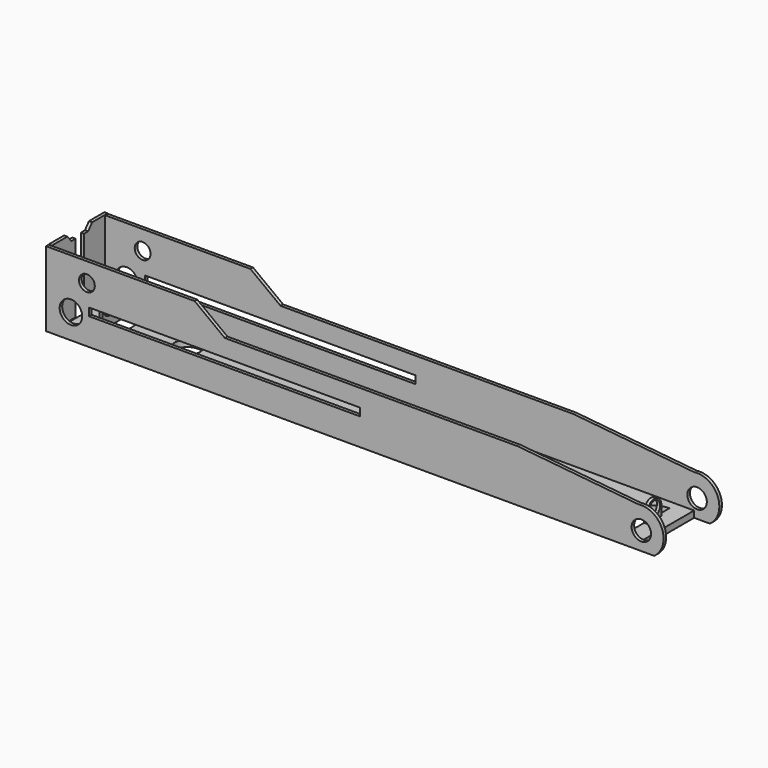
from build123d import *

# Parameters (mm, degrees)
F0_R      = 1.75
F0_R_2    = 1.51
F0_R_3    = 1.225
F8_DEPTH  = 0.5
F2_R      = 1.75
F2_R_2    = 1.51
F2_R_3    = 1.225
F9_DEPTH  = 0.5
F7_R      = 1.97
F10_DEPTH = 0.5
F11_DEPTH = 1
F12_DEPTH = 0.5
F13_DEPTH = 25
F16_DEPTH = 0.5
F17_DEPTH = 0.5
F18_W     = 41.976
F18_H     = 1.2
F19_DEPTH = 11.301


# Not quite as in the source:
# - a feature names something its author has since deleted; it is built from what else it names


with BuildPart() as f8:
    # F0 (on Front) → F8 (new body)
    with BuildSketch(Plane.XZ):
        with BuildLine():
            Line((-24.095, 11.6), (-47.125, 11.6))
            Line((-47.125, 11.6), (-47.125, 0))
            Line((-47.125, 0), (47.125, 0))
            ThreePointArc((47.125, 0), (48.3457892371, 4.0785044966), (44.6764603032, 6.2373353065))
            Line((44.6764603032, 6.2373353065), (25.9870177338, 8.0793821146))
            Line((25.9870177338, 8.0793821146), (-19.4229822662, 8.0793821146))
            Line((-19.4229822662, 8.0793821146), (-24.095, 11.6))
        make_face()
        with Locations((-43.275, 3.85)):
            Circle(F0_R, mode=Mode.SUBTRACT)
        with Locations((45.1343327214, 2.8178092836)):
            Circle(F0_R_2, mode=Mode.SUBTRACT)
        with Locations((-40.8, 8.615)):
            Circle(F0_R_3, mode=Mode.SUBTRACT)
    extrude(amount=F8_DEPTH)

    # F6 (on offset) → F9, piece 2 (join)
    with BuildSketch(Plane.YZ.offset(-47.125)):
        Polygon((3.7804580054, 10.7198863682), (3, 11.65), (0, 11.65), (0, 0), (4.5804580054, 0), (4.5804580054, 10.7198863682), align=None)
    extrude(amount=F9_DEPTH)



with BuildPart() as f8b:
    # F2 (on offset) → F8, piece 2 (new body)
    with BuildSketch(Plane.XZ.offset(-10.8)):
        with BuildLine():
            Line((-19.4229822662, 8.0793821146), (-24.095, 11.6))
            Line((-24.095, 11.6), (-47.125, 11.6))
            Line((-47.125, 11.6), (-47.125, 0))
            Line((-47.125, 0), (47.125, 0))
            ThreePointArc((47.125, 0), (48.3457892371, 4.0785044966), (44.6764603032, 6.2373353065))
            Line((44.6764603032, 6.2373353065), (25.9870177338, 8.0793821146))
            Line((25.9870177338, 8.0793821146), (-19.4229822662, 8.0793821146))
        make_face()
        with Locations((-43.275, 3.85)):
            Circle(F2_R, mode=Mode.SUBTRACT)
        with Locations((45.1343327214, 2.8178092836)):
            Circle(F2_R_2, mode=Mode.SUBTRACT)
        with Locations((-40.8, 8.615)):
            Circle(F2_R_3, mode=Mode.SUBTRACT)
    extrude(amount=F8_DEPTH)

    # F6 (on offset) → F9 (join)
    with BuildSketch(Plane.YZ.offset(-47.125)):
        Polygon((10.8, 0), (10.8, 11.65), (7.8, 11.65), (7.0195419946, 10.7198863682), (6.2195419946, 10.7198863682), (6.2195419946, 0), align=None)
    extrude(amount=F9_DEPTH)


with BuildPart() as f8_1:
    add(f8.part)

    add(f8b.part)  # F10 merges F8b
    # F7 (on Top) → F10 (join)
    with BuildSketch(Plane.XY):
        Polygon((-47.125, 4.45), (-47.125, 0), (-46.325, 0), (-46.325, 1.5), (-45.2581904829, 1.5), (-45.2581904829, 9.3), (-46.325, 9.3), (-46.325, 10.8), (-47.125, 10.8), (-47.125, 5.95), align=None)
        Polygon((-46.325, 1.5), (-46.325, 0), (-24.095, 0), (-19.4229822662, 0), (25.9870177338, 0), (44.676, 0), (44.676, 10.8), (25.9870177338, 10.8), (-19.4229822662, 10.8), (-46.325, 10.8), (-46.325, 9.3), (-45.2581904829, 9.3), (-45.2581904829, 1.5), align=None)
        with BuildLine():
            Line((-41.976, 1.89), (-41.976, 8.91))
            ThreePointArc((-41.976, 8.91), (-38.466, 5.4), (-41.976, 1.89))
        make_face(mode=Mode.SUBTRACT)
        with Locations((-29.946, 5.4)):
            Circle(F7_R, mode=Mode.SUBTRACT)
        with Locations((29.946, 5.4)):
            Circle(F7_R, mode=Mode.SUBTRACT)
        with BuildLine():
            Line((41.976, 8.91), (41.976, 1.89))
            ThreePointArc((41.976, 1.89), (38.466, 5.4), (41.976, 8.91))
        make_face(mode=Mode.SUBTRACT)
    extrude(amount=F10_DEPTH)

    # F7 (on Top) → F11 (join)
    with BuildSketch(Plane.XY):
        Polygon((-46.325, 1.5), (-46.325, 0), (-24.095, 0), (-19.4229822662, 0), (25.9870177338, 0), (44.676, 0), (44.676, 10.8), (25.9870177338, 10.8), (-19.4229822662, 10.8), (-46.325, 10.8), (-46.325, 9.3), (-45.2581904829, 9.3), (-45.2581904829, 1.5), align=None)
        with BuildLine():
            Line((-41.976, 1.89), (-41.976, 8.91))
            ThreePointArc((-41.976, 8.91), (-38.466, 5.4), (-41.976, 1.89))
        make_face(mode=Mode.SUBTRACT)
        with Locations((-29.946, 5.4)):
            Circle(F7_R, mode=Mode.SUBTRACT)
        with Locations((29.946, 5.4)):
            Circle(F7_R, mode=Mode.SUBTRACT)
        with BuildLine():
            Line((41.976, 8.91), (41.976, 1.89))
            ThreePointArc((41.976, 1.89), (38.466, 5.4), (41.976, 8.91))
        make_face(mode=Mode.SUBTRACT)
    extrude(amount=F11_DEPTH)

    # F6 (on offset) → F12 (join)
    with BuildSketch(Plane.YZ.offset(-47.125)):
        Polygon((3.7804580054, 10.7198863682), (3, 11.65), (0, 11.65), (0, 0), (4.5804580054, 0), (4.5804580054, 10.7198863682), align=None)
    extrude(amount=F12_DEPTH)

    # F13 (cut): a face of the model
    f13_faces = [f8_1.faces().sort_by_distance(p)[0] for p in [
        (-46.0368491628, 5.3368390391, 0.5),
    ]]
    extrude(f13_faces, amount=-F13_DEPTH, mode=Mode.SUBTRACT)

    # F14 (on face) → F16 (join)
    with BuildSketch(Plane.YZ.offset(-41.976)):
        with BuildLine():
            Line((4, 2.55), (4, 1))
            Line((4, 1), (4.5804580054, 1))
            Line((4.5804580054, 1), (4.5804580054, 1.7362401346))
            ThreePointArc((4.5804580054, 1.7362401346), (4.23, 2.55), (4.5804580054, 3.3637598654))
            Line((4.5804580054, 3.3637598654), (4.5804580054, 3.6591912001))
            ThreePointArc((4.5804580054, 3.6591912001), (4.1538851032, 3.175946606), (4, 2.55))
        make_face()
        with BuildLine():
            ThreePointArc((6.2195419946, 3.5826648631), (5.4129608614, 3.8985310267), (4.5804580054, 3.6591912001))
            Line((4.5804580054, 3.6591912001), (4.5804580054, 3.3637598654))
            ThreePointArc((4.5804580054, 3.3637598654), (5.4235415848, 3.6675829434), (6.2195419946, 3.2559013526))
            Line((6.2195419946, 3.2559013526), (6.2195419946, 3.5826648631))
        make_face()
        with BuildLine():
            Line((4.5804580054, 1.7362401346), (4.5804580054, 1))
            Line((4.5804580054, 1), (6.2195419946, 1))
            Line((6.2195419946, 1), (6.2195419946, 1.8440986474))
            ThreePointArc((6.2195419946, 1.8440986474), (5.4235415848, 1.4324170566), (4.5804580054, 1.7362401346))
        make_face()
        with BuildLine():
            Line((6.2195419946, 1.8440986474), (6.2195419946, 1))
            Line((6.2195419946, 1), (6.7, 1))
            Line((6.7, 1), (6.7, 2.55))
            ThreePointArc((6.7, 2.55), (6.5740060647, 3.1194814779), (6.2195419946, 3.5826648631))
            Line((6.2195419946, 3.5826648631), (6.2195419946, 3.2559013526))
            ThreePointArc((6.2195419946, 3.2559013526), (6.4055299697, 2.9245083217), (6.47, 2.55))
            ThreePointArc((6.47, 2.55), (6.4055299697, 2.1754916783), (6.2195419946, 1.8440986474))
        make_face()
    extrude(amount=-F16_DEPTH)

    # F15 (on face) → F17 (join)
    with BuildSketch(Plane(origin=(41.976, 0, 0), x_dir=(0, -1, 0), z_dir=(-1, 0, 0))):
        with BuildLine():
            ThreePointArc((-4.5804580054, 3.3637598654), (-4.23, 2.55), (-4.5804580054, 1.7362401346))
            Line((-4.5804580054, 1.7362401346), (-4.5804580054, 1))
            Line((-4.5804580054, 1), (-4, 1))
            Line((-4, 1), (-4, 2.55))
            ThreePointArc((-4, 2.55), (-4.1538851032, 3.175946606), (-4.5804580054, 3.6591912001))
            Line((-4.5804580054, 3.6591912001), (-4.5804580054, 3.3637598654))
        make_face()
        with BuildLine():
            Line((-6.2195419946, 3.5826648631), (-6.2195419946, 3.2559013526))
            ThreePointArc((-6.2195419946, 3.2559013526), (-5.4235415848, 3.6675829434), (-4.5804580054, 3.3637598654))
            Line((-4.5804580054, 3.3637598654), (-4.5804580054, 3.6591912001))
            ThreePointArc((-4.5804580054, 3.6591912001), (-5.4129608614, 3.8985310267), (-6.2195419946, 3.5826648631))
        make_face()
        with BuildLine():
            Line((-6.2195419946, 1), (-6.2195419946, 1.8440986474))
            ThreePointArc((-6.2195419946, 1.8440986474), (-6.47, 2.55), (-6.2195419946, 3.2559013526))
            Line((-6.2195419946, 3.2559013526), (-6.2195419946, 3.5826648631))
            ThreePointArc((-6.2195419946, 3.5826648631), (-6.5740060647, 3.1194814779), (-6.7, 2.55))
            Line((-6.7, 2.55), (-6.7, 1))
            Line((-6.7, 1), (-6.2195419946, 1))
        make_face()
        with BuildLine():
            ThreePointArc((-4.5804580054, 1.7362401346), (-5.4235415848, 1.4324170566), (-6.2195419946, 1.8440986474))
            Line((-6.2195419946, 1.8440986474), (-6.2195419946, 1))
            Line((-6.2195419946, 1), (-4.5804580054, 1))
            Line((-4.5804580054, 1), (-4.5804580054, 1.7362401346))
        make_face()
    extrude(amount=-F17_DEPTH)

    # F18 (on face) → F19 (cut, through all)
    with BuildSketch(Plane.XZ.offset(0.5)):
        with Locations((-19.4615396968, 4.8)):
            Rectangle(F18_W, F18_H)
    extrude(amount=-F19_DEPTH, mode=Mode.SUBTRACT)


solid = f8_1.part
